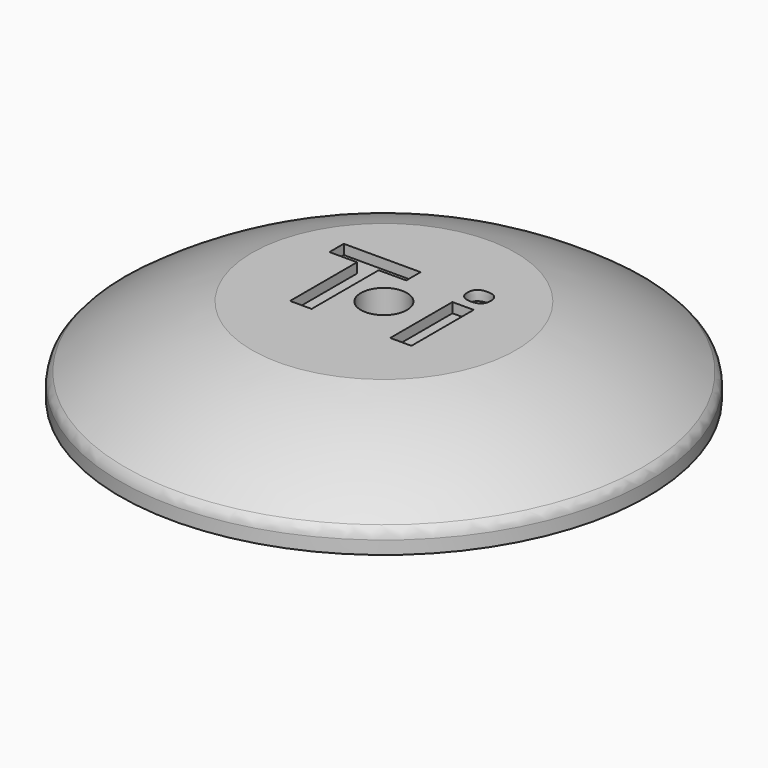
from build123d import *

# Parameters (mm, degrees)
F2_TEXT_SIZE = 21.5960466044
F3_DEPTH     = 1.5
F4_SIZE      = 1
F5_R         = 3.5
F6_DEPTH     = 13.001
F7_R         = 2


# Not quite as in the source:
# - Text() gives the source's letters only with a copy of the font that has no kerning and outlines rounded to 1/6400 em; it was checked with that copy


with BuildPart() as f1:
    # F0 (on Front) → F1 (revolve)
    with BuildSketch(Plane.XZ):
        with BuildLine():
            Line((-5.9, 0), (0, 0))
            Line((0, 0), (0, 13))
            Line((0, 13), (-20, 13))
            ThreePointArc((-20, 13), (-30.4699630771, 8.9399261541), (-40, 3))
            Line((-40, 3), (-40, 0))
            Line((-40, 0), (-20.4, 10))
            Line((-20.4, 10), (-5.9, 10))
            Line((-5.9, 10), (-5.9, 0))
        make_face()
    revolve(axis=Axis((0, 0, 6.5), (0, 0, 1)))

    # F2 (on face) → F3 (cut)
    with BuildSketch(Plane.XY.offset(13)):
        with Locations((-13.3846257813, -6.8317162804)):
            Text('T i', F2_TEXT_SIZE, font='Open Sans', font_style=FontStyle.BOLD, text_align=(TextAlign.LEFT, TextAlign.BOTTOM))
    extrude(amount=-F3_DEPTH, mode=Mode.SUBTRACT)

    # F4
    f4_edges = [f1.edges().sort_by_distance(p)[0] for p in [
        (5.9, 0, 0),
    ]]
    chamfer(f4_edges, length=F4_SIZE)

    # F5 (on face) → F6 (cut, through all)
    with BuildSketch(Plane.XY.offset(13)):
        Circle(F5_R)
    extrude(amount=-F6_DEPTH, mode=Mode.SUBTRACT)

    # F7
    f7_edges = [f1.edges().sort_by_distance(p)[0] for p in [
        (40, 0, 3),
    ]]
    fillet(f7_edges, radius=F7_R)


solid = f1.part
